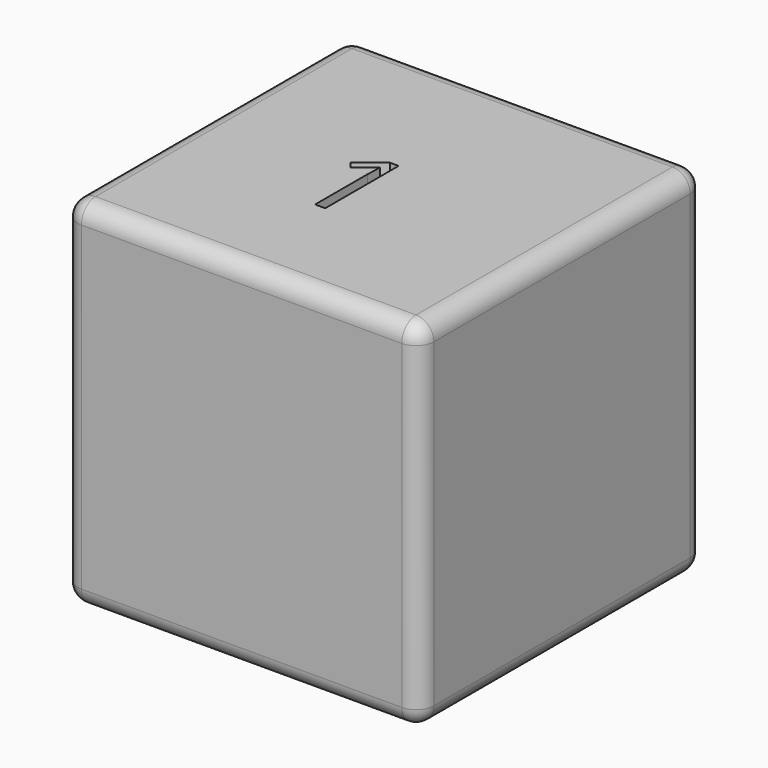
from build123d import *

# Parameters (mm, degrees)
F0_W         = 100
F0_H         = 100
F1_DEPTH     = 100
F2_R         = 5
F3_TEXT_SIZE = 36.084816222
F4_DEPTH     = 12
F5_TEXT_SIZE = 36.7878373557
F6_DEPTH     = 12
F7_TEXT_SIZE = 26.4903064817
F8_DEPTH     = 12
F9_TEXT_SIZE = 50.9516232544
F10_DEPTH    = 12


# Not quite as in the source:
# - Text() gives the source's letters only with a copy of the font that has no kerning and outlines rounded to 1/6400 em; it was checked with that copy


with BuildPart() as f1:
    # F0 (on Top) → F1 (new body)
    with BuildSketch(Plane.XY):
        Rectangle(F0_W, F0_H)
    extrude(amount=F1_DEPTH)

    # F2
    f2_edges = [f1.edges().sort_by_distance(p)[0] for p in [
        (-50, 0, 100),
        (0, 50, 100),
        (50, 0, 100),
        (0, -50, 100),
        (-50, -50, 50),
        (-50, 50, 50),
        (-50, 0, 0),
        (50, 50, 50),
        (0, 50, 0),
        (50, -50, 50),
        (50, 0, 0),
        (0, -50, 0),
    ]]
    fillet(f2_edges, radius=F2_R)

    # F3 (on face) → F4 (cut)
    with BuildSketch(Plane.XY.offset(100)):
        with Locations((-14.8070314899, -17.8622826934)):
            Text('1', F3_TEXT_SIZE, font='Open Sans', text_align=(TextAlign.LEFT, TextAlign.BOTTOM))
    extrude(amount=-F4_DEPTH, mode=Mode.SUBTRACT)

    # F5 (on face) → F6 (cut)
    with BuildSketch(Plane(origin=(0, 0, 0), x_dir=(1, 0, 0), z_dir=(0, 0, -1))):
        with Locations((-6.6652959213, -20.0272332877)):
            Text('1', F5_TEXT_SIZE, font='Open Sans', text_align=(TextAlign.LEFT, TextAlign.BOTTOM))
    extrude(amount=-F6_DEPTH, mode=Mode.SUBTRACT)

    # F7 (on face) → F8 (cut)
    with BuildSketch(Plane(origin=(0, 50, 0), x_dir=(-1, 0, 0), z_dir=(0, 1, 0))):
        with Locations((-12.0264086872, 43.5306318104)):
            Text('1', F7_TEXT_SIZE, font='Open Sans', text_align=(TextAlign.LEFT, TextAlign.BOTTOM))
    extrude(amount=F8_DEPTH, mode=Mode.SUBTRACT)

    # F9 (on face) → F10 (cut)
    with BuildSketch(Plane(origin=(0, 50, 0), x_dir=(-1, 0, 0), z_dir=(0, 1, 0))):
        with Locations((-16.2007175386, 33.2125350833)):
            Text('1', F9_TEXT_SIZE, font='Open Sans', text_align=(TextAlign.LEFT, TextAlign.BOTTOM))
    extrude(amount=-F10_DEPTH, mode=Mode.SUBTRACT)


solid = f1.part
